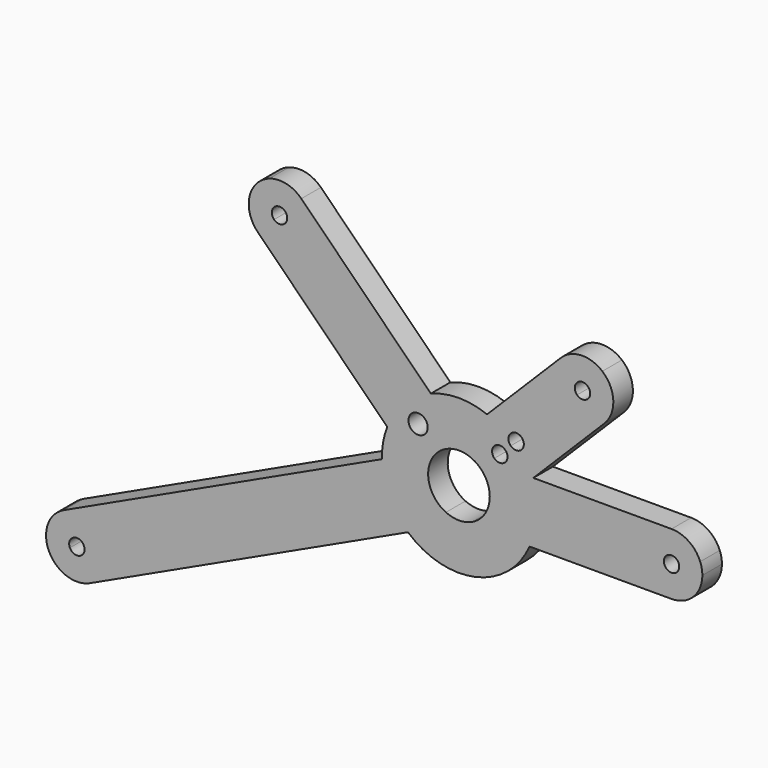
from build123d import *

# Parameters (mm, degrees)
F1_DEPTH = 3.175


# Not quite as in the source:
# - a length typed as a fraction of an inch, garbled in the dataset ("3 / 203.2 mm" for 3/8 in), is restored
# - a feature names something its author has since deleted; it is built from what else it names


with BuildPart() as f1:
    # F0 (on Front) → F1 (new body)
    with BuildSketch(Plane.XZ):
        with BuildLine():
            ThreePointArc((41.6017871916, 14.91), (41.5307431297, 15.6605366323), (41.3201345734, 16.3844126791))
            ThreePointArc((41.3201345734, 16.3844126791), (39.8492690362, 18.218900929), (37.6017871916, 18.91))
            Line((37.6017871916, 18.91), (19.6568542495, 18.91))
            Line((19.6568542495, 18.91), (28.870343186, 28.1234889365))
            ThreePointArc((28.870343186, 28.1234889365), (30.0382240231, 31.1237376944), (28.617137145, 34.0126735442))
            ThreePointArc((28.617137145, 34.0126735442), (25.870094428, 34.9482240231), (23.2134889365, 33.780343186))
            Line((23.2134889365, 33.780343186), (13.6523135737, 24.2191678232))
            ThreePointArc((13.6523135737, 24.2191678232), (10, 24.91), (6.3476864263, 24.2191678232))
            Line((6.3476864263, 24.2191678232), (-10.4648587405, 41.03171299))
            ThreePointArc((-10.4648587405, 41.03171299), (-12.3998071782, 42.1022210835), (-14.6078257676, 41.9811139245))
            ThreePointArc((-14.6078257676, 41.9811139245), (-15.418464559, 41.5920342359), (-16.12171299, 41.03171299))
            ThreePointArc((-16.12171299, 41.03171299), (-17.2932858653, 38.2032858653), (-16.12171299, 35.3748587405))
            Line((-16.12171299, 35.3748587405), (0.6908321768, 18.5623135737))
            ThreePointArc((0.6908321768, 18.5623135737), (0.1519224699, 16.6464817767), (0.003078879, 14.6618707992))
            Line((0.003078879, 14.6618707992), (-41.296146258, -4.5962741581))
            ThreePointArc((-41.296146258, -4.5962741581), (-43.1811508594, -6.4281956325), (-43.5221795995, -9.0345106623))
            ThreePointArc((-43.5221795995, -9.0345106623), (-43.4019791332, -9.4816883664), (-43.2309043592, -9.9119783532))
            ThreePointArc((-43.2309043592, -9.9119783532), (-40.9737537843, -11.9802757894), (-37.9152001641, -11.8467364544))
            Line((-37.9152001641, -11.8467364544), (3.3840249729, 7.4114085029))
            ThreePointArc((3.3840249729, 7.4114085029), (12.1643961394, 5.1470399288), (19.1651513899, 10.91))
            Line((19.1651513899, 10.91), (37.6017871916, 10.91))
            ThreePointArc((37.6017871916, 10.91), (40.4302143163, 12.0815728753), (41.6017871916, 14.91))
        make_face()
        with BuildLine():
            ThreePointArc((-40.5119809981, -8.644123568), (-40.5453658318, -7.8794851629), (-40.0282914728, -7.3151975192))
            ThreePointArc((-40.0282914728, -7.3151975192), (-39.2636530677, -7.2818126855), (-38.699365424, -7.7988870445))
            ThreePointArc((-38.699365424, -7.7988870445), (-38.6293772039, -8.0050656923), (-38.605673211, -8.2215053062))
            ThreePointArc((-38.605673211, -8.2215053062), (-38.7622817652, -8.7588049146), (-39.1830549493, -9.1278130933))
            ThreePointArc((-39.1830549493, -9.1278130933), (-39.9476933544, -9.161197927), (-40.5119809981, -8.644123568))
        make_face(mode=Mode.SUBTRACT)
        with BuildLine():
            ThreePointArc((-12.2932858653, 38.2032858653), (-12.3694063328, 37.8206024329), (-12.5861790841, 37.4961790841))
            ThreePointArc((-12.5861790841, 37.4961790841), (-13.2932858653, 37.2032858653), (-14.0003926465, 37.4961790841))
            ThreePointArc((-14.0003926465, 37.4961790841), (-14.2932858653, 38.2032858653), (-14.0003926465, 38.9103926465))
            ThreePointArc((-14.0003926465, 38.9103926465), (-13.2932858653, 39.2032858653), (-12.5861790841, 38.9103926465))
            ThreePointArc((-12.5861790841, 38.9103926465), (-12.3694063328, 38.5859692976), (-12.2932858653, 38.2032858653))
        make_face(mode=Mode.SUBTRACT)
        with BuildLine():
            ThreePointArc((14, 14.91), (13.3735657833, 12.7608015666), (11.690473047, 11.2847688519))
            ThreePointArc((11.690473047, 11.2847688519), (10, 10.91), (8.309526953, 11.2847688519))
            ThreePointArc((8.309526953, 11.2847688519), (6.060768988, 14.2154072893), (7.1715728753, 17.7384271247))
            ThreePointArc((7.1715728753, 17.7384271247), (10, 18.91), (12.8284271247, 17.7384271247))
            ThreePointArc((12.8284271247, 17.7384271247), (13.69551813, 16.4407337295), (14, 14.91))
        make_face(mode=Mode.SUBTRACT)
        with BuildLine():
            ThreePointArc((5.9466991411, 20.2133008589), (5.8515485567, 19.7349465684), (5.5805826176, 19.3294173824))
            ThreePointArc((5.5805826176, 19.3294173824), (3.8128156646, 19.3294173824), (3.8128156646, 21.0971843354))
            ThreePointArc((3.8128156646, 21.0971843354), (5.1750534316, 21.3681502745), (5.9466991411, 20.2133008589))
        make_face(mode=Mode.SUBTRACT)
        with BuildLine():
            ThreePointArc((16.3033008589, 20.2133008589), (15.6859842913, 19.2894213264), (14.5961940777, 19.5061940777))
            ThreePointArc((14.5961940777, 19.5061940777), (14.5961940777, 20.9204076401), (16.0104076401, 20.9204076401))
            ThreePointArc((16.0104076401, 20.9204076401), (16.2271803914, 20.5959842913), (16.3033008589, 20.2133008589))
        make_face(mode=Mode.SUBTRACT)
        with BuildLine():
            ThreePointArc((36.6017871916, 14.91), (37.6017871916, 15.91), (38.6017871916, 14.91))
            ThreePointArc((38.6017871916, 14.91), (37.6017871916, 13.91), (36.6017871916, 14.91))
        make_face(mode=Mode.SUBTRACT)
        with BuildLine():
            ThreePointArc((18.4246212025, 22.3346212025), (17.8073046348, 21.4107416699), (16.7175144213, 21.6275144213))
            ThreePointArc((16.7175144213, 21.6275144213), (16.7175144213, 23.0417279836), (18.1317279836, 23.0417279836))
            ThreePointArc((18.1317279836, 23.0417279836), (18.348500735, 22.7173046348), (18.4246212025, 22.3346212025))
        make_face(mode=Mode.SUBTRACT)
        with BuildLine():
            ThreePointArc((26.7490228424, 30.24480928), (26.0419160612, 29.9519160612), (25.33480928, 30.24480928))
            ThreePointArc((25.33480928, 30.24480928), (25.0419160612, 30.9519160612), (25.33480928, 31.6590228424))
            ThreePointArc((25.33480928, 31.6590228424), (26.0419160612, 31.9519160612), (26.7490228424, 31.6590228424))
            ThreePointArc((26.7490228424, 31.6590228424), (26.9657955937, 31.3345994936), (27.0419160612, 30.9519160612))
            ThreePointArc((27.0419160612, 30.9519160612), (26.9657955937, 30.5692326289), (26.7490228424, 30.24480928))
        make_face(mode=Mode.SUBTRACT)
    extrude(amount=F1_DEPTH)


solid = f1.part
